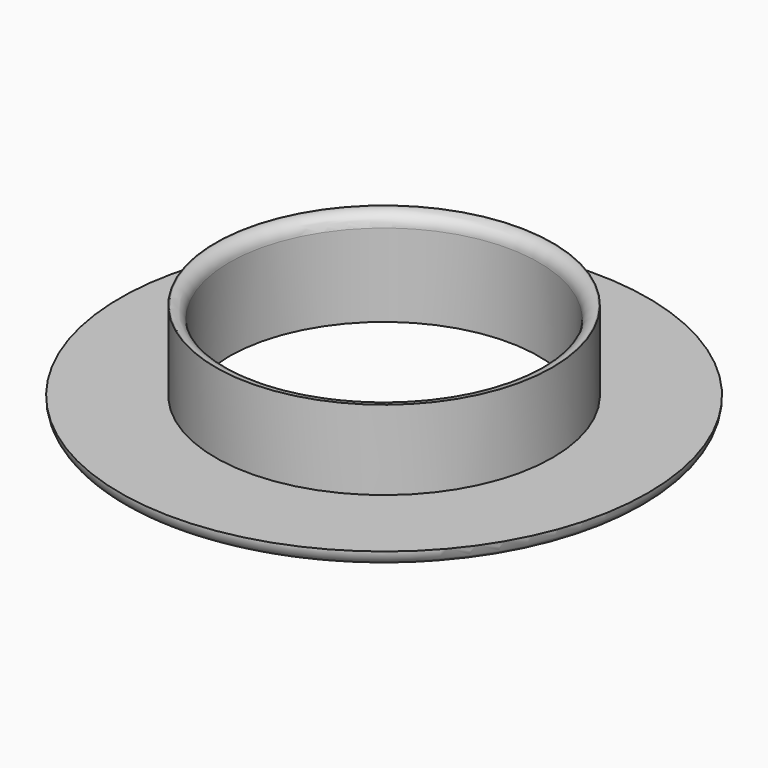
from build123d import *

# Parameters (mm, degrees)
F0_R     = 41.5
F0_R_2   = 26.5
F1_DEPTH = 2.5
F0_R_3   = 24.35
F2_DEPTH = 15
F3_R     = 2.49999
F4_R     = 2


# Not quite as in the source:
# - a fillet or chamfer is up to 0.001 mm smaller than in the source, because OpenCascade refuses the exact size


with BuildPart() as f1:
    # F0 (on Top) → F1 (new body)
    with BuildSketch(Plane.XY):
        Circle(F0_R)
        Circle(F0_R_2, mode=Mode.SUBTRACT)
    extrude(amount=F1_DEPTH)

    # F0 (on Top) → F2 (join)
    with BuildSketch(Plane.XY):
        Circle(F0_R_2)
        Circle(F0_R_3, mode=Mode.SUBTRACT)
    extrude(amount=F2_DEPTH)

    # F3 (radius 2.5 in the source; OpenCascade refuses exactly that, so slightly less here)
    f3_edges = [f1.edges().sort_by_distance(p)[0] for p in [
        (-41.5, 0, 0),
    ]]
    fillet(f3_edges, radius=F3_R)

    # F4
    f4_edges = [f1.edges().sort_by_distance(p)[0] for p in [
        (-24.35, 0, 15),
    ]]
    fillet(f4_edges, radius=F4_R)


solid = f1.part
